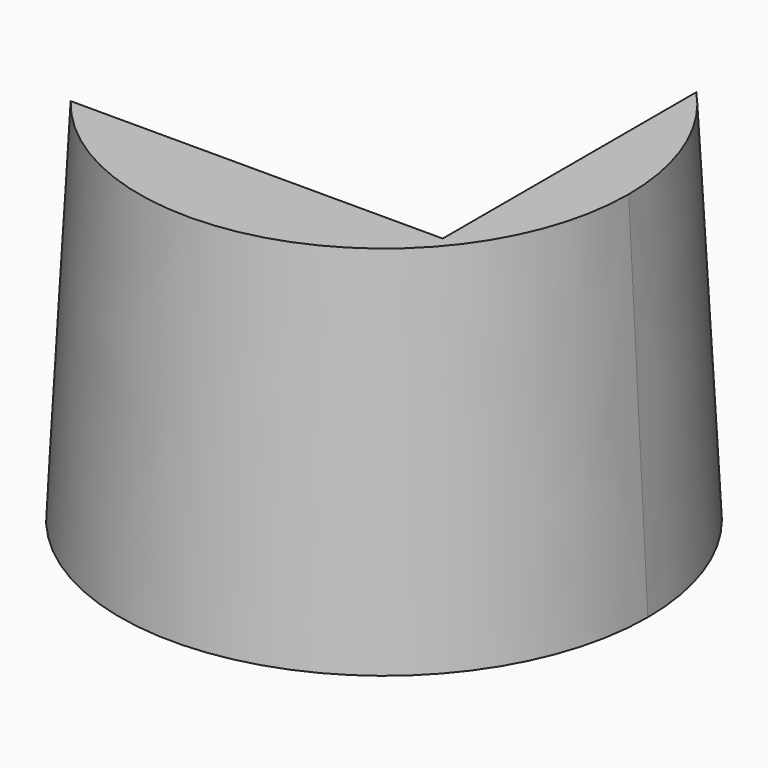
from build123d import *

# Parameters (mm, degrees)
F1_DEPTH               = 45.212
DRAFT_F1_DRAFTED_ANGLE = -3


# Not quite as in the source:
# - an extrude with a draft is written as a straight extrude whose walls are then drafted


with BuildPart() as f1:
    # F0 (on Top) → F1 (new body)
    with BuildSketch(Plane.XY):
        with BuildLine():
            Line((21.9891462475, 6.060283654), (21.9891462475, -33.0825895071))
            Line((21.9891462475, -33.0825895071), (-23.9528412618, -33.0825895071))
            ThreePointArc((-23.9528412618, -33.0825895071), (9.7273690765, -43.2708542465), (30.2158852455, -14.6635472775))
            ThreePointArc((30.2158852455, -14.6635472775), (28.083992245, -3.5150451021), (21.9891462475, 6.060283654))
        make_face()
    extrude(amount=-F1_DEPTH)

    # draft_F1_drafted
    draft_f1_drafted_walls = [f1.faces().sort_by_distance(p)[0] for p in [
        (19.5960494578, -37.6634291644, -30.1413333333),
        (21.9891462475, -13.5111529266, -30.1413333333),
        (-0.9818475071, -33.0825895071, -30.1413333333),
    ]]
    draft(draft_f1_drafted_walls, neutral_plane=Plane(origin=(0, 0, 0), x_dir=(1, 0, 0), z_dir=(0, 0, -1)), angle=DRAFT_F1_DRAFTED_ANGLE)


solid = f1.part
